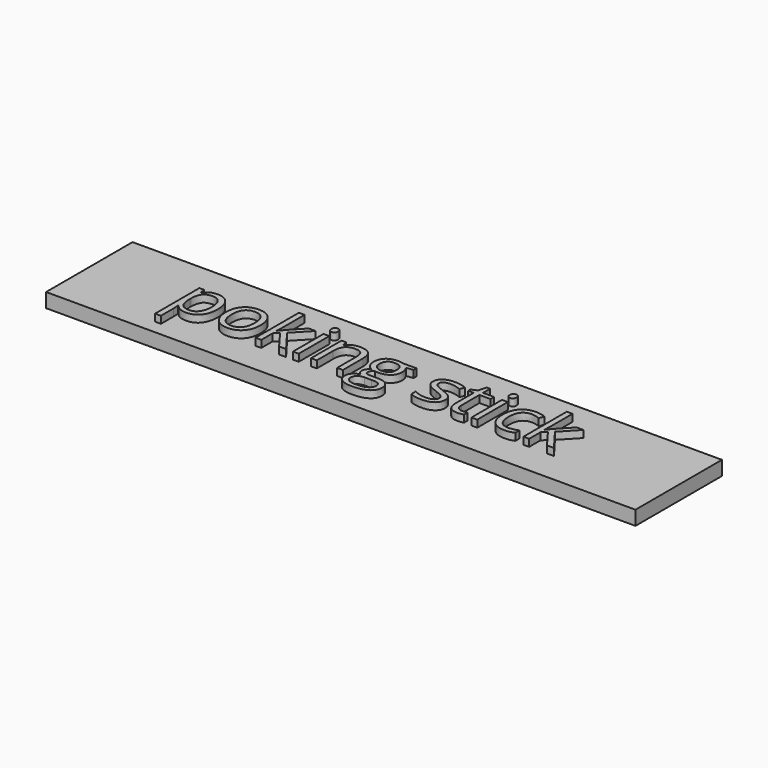
from build123d import *

# Parameters (mm, degrees)
F0_W         = 105.0174571574
F0_H         = 19.2578183487
F0_W_2       = 1.0298908098
F0_H_2       = 6.7964855942
F1_DEPTH     = 2.54
F0_TEXT_SIZE = 12.7000022783
F2_DEPTH     = 3.81


# Not quite as in the source:
# - Text() gives the source's letters only with a copy of the font that has no kerning and outlines rounded to 1/6400 em; it was checked with that copy


with BuildPart() as f1:
    # F0 (on Top) → F1 (new body)
    with BuildSketch(Plane.XY):
        with Locations((9.0054553002, 18.7729089521)):
            Rectangle(F0_W, F0_H)
        with BuildLine():
            add(Edge.make_bspline(
                [(-20.8257423863, 15.4884978257), (-21.5728597078, 14.5608023468), (-22.900406821, 14.5608023468)],
                knots=[0, 0, 0, 1, 1, 1], degree=2))
            add(Edge.make_bspline(
                [(-22.900406821, 14.5608023468), (-23.5651725652, 14.5608023468), (-24.1138523511, 14.8058727032)],
                knots=[0, 0, 0, 1, 1, 1], degree=2))
            add(Edge.make_bspline(
                [(-24.1138523511, 14.8058727032), (-24.6625321371, 15.0509430597), (-25.0336103286, 15.5609275262)],
                knots=[0, 0, 0, 1, 1, 1], degree=2))
            Line((-25.0336103286, 15.5609275262), (-25.1090165922, 15.5609275262))
            add(Edge.make_bspline(
                [(-25.1090165922, 15.5609275262), (-25.0336103286, 14.9656149194), (-25.0336103286, 14.4318179486)],
                knots=[0, 0, 0, 1, 1, 1], degree=2))
            Line((-25.0336103286, 14.4318179486), (-25.0336103286, 11.6338486967))
            Line((-25.0336103286, 11.6338486967), (-26.0635011384, 11.6338486967))
            Line((-26.0635011384, 11.6338486967), (-26.0635011384, 21.4823035884))
            Line((-26.0635011384, 21.4823035884), (-25.2260947382, 21.4823035884))
            Line((-25.2260947382, 21.4823035884), (-25.0832197125, 20.5516315465))
            Line((-25.0832197125, 20.5516315465), (-25.0336103286, 20.5516315465))
            add(Edge.make_bspline(
                [(-25.0336103286, 20.5516315465), (-24.6367352574, 21.1112253969), (-24.1098836004, 21.3592723164)],
                knots=[0, 0, 0, 1, 1, 1], degree=2))
            add(Edge.make_bspline(
                [(-24.1098836004, 21.3592723164), (-23.5830319434, 21.6073192359), (-22.900406821, 21.6073192359)],
                knots=[0, 0, 0, 1, 1, 1], degree=2))
            add(Edge.make_bspline(
                [(-22.900406821, 21.6073192359), (-21.5490472035, 21.6073192359), (-20.8138361341, 20.68260032)],
                knots=[0, 0, 0, 1, 1, 1], degree=2))
            add(Edge.make_bspline(
                [(-20.8138361341, 20.68260032), (-20.0786250647, 19.7578814041), (-20.0786250647, 18.091006105)],
                knots=[0, 0, 0, 1, 1, 1], degree=2))
            add(Edge.make_bspline(
                [(-20.0786250647, 18.091006105), (-20.0786250647, 16.4161933046), (-20.8257423863, 15.4884978257)],
                knots=[0, 0, 0, 1, 1, 1], degree=2))
        make_face(mode=Mode.SUBTRACT)
        with BuildLine():
            add(Edge.make_bspline(
                [(-13.2553504032, 20.657795628), (-12.4149674399, 19.7082720202), (-12.4149674399, 18.091006105)],
                knots=[0, 0, 0, 1, 1, 1], degree=2))
            add(Edge.make_bspline(
                [(-12.4149674399, 18.091006105), (-12.4149674399, 16.4280995567), (-13.2513816525, 15.4944509517)],
                knots=[0, 0, 0, 1, 1, 1], degree=2))
            add(Edge.make_bspline(
                [(-13.2513816525, 15.4944509517), (-14.087795865, 14.5608023468), (-15.5641711299, 14.5608023468)],
                knots=[0, 0, 0, 1, 1, 1], degree=2))
            add(Edge.make_bspline(
                [(-15.5641711299, 14.5608023468), (-16.4769837936, 14.5608023468), (-17.1834214204, 14.9894274236)],
                knots=[0, 0, 0, 1, 1, 1], degree=2))
            add(Edge.make_bspline(
                [(-17.1834214204, 14.9894274236), (-17.8898590471, 15.4180525005), (-18.2748278662, 16.217755769)],
                knots=[0, 0, 0, 1, 1, 1], degree=2))
            add(Edge.make_bspline(
                [(-18.2748278662, 16.217755769), (-18.6597966852, 17.0174590375), (-18.6597966852, 18.091006105)],
                knots=[0, 0, 0, 1, 1, 1], degree=2))
            add(Edge.make_bspline(
                [(-18.6597966852, 18.091006105), (-18.6597966852, 19.751928278), (-17.8283434111, 20.6796237569)],
                knots=[0, 0, 0, 1, 1, 1], degree=2))
            add(Edge.make_bspline(
                [(-17.8283434111, 20.6796237569), (-16.9968901369, 21.6073192359), (-15.520514872, 21.6073192359)],
                knots=[0, 0, 0, 1, 1, 1], degree=2))
            add(Edge.make_bspline(
                [(-15.520514872, 21.6073192359), (-14.0957333665, 21.6073192359), (-13.2553504032, 20.657795628)],
                knots=[0, 0, 0, 1, 1, 1], degree=2))
        make_face(mode=Mode.SUBTRACT)
        with Locations((-3.4287236404, 18.0840607913)):
            Rectangle(F0_W_2, F0_H_2, mode=Mode.SUBTRACT)
        with BuildLine():
            Line((4.9503013003, 14.6858179942), (3.9204104905, 14.6858179942))
            Line((3.9204104905, 14.6858179942), (3.9204104905, 19.083193783))
            add(Edge.make_bspline(
                [(3.9204104905, 19.083193783), (3.9204104905, 19.9126626818), (3.5423869852, 20.3224361929)],
                knots=[0, 0, 0, 1, 1, 1], degree=2))
            add(Edge.make_bspline(
                [(3.5423869852, 20.3224361929), (3.1643634799, 20.7322097039), (2.35672271, 20.7322097039)],
                knots=[0, 0, 0, 1, 1, 1], degree=2))
            add(Edge.make_bspline(
                [(2.35672271, 20.7322097039), (1.2911131439, 20.7322097039), (0.7950193049, 20.155748663)],
                knots=[0, 0, 0, 1, 1, 1], degree=2))
            add(Edge.make_bspline(
                [(0.7950193049, 20.155748663), (0.2989254659, 19.579287622), (0.2989254659, 18.2517405089)],
                knots=[0, 0, 0, 1, 1, 1], degree=2))
            Line((0.2989254659, 18.2517405089), (0.2989254659, 14.6858179942))
            Line((0.2989254659, 14.6858179942), (-0.7309653439, 14.6858179942))
            Line((-0.7309653439, 14.6858179942), (-0.7309653439, 21.4823035884))
            Line((-0.7309653439, 21.4823035884), (0.1064410563, 21.4823035884))
            Line((0.1064410563, 21.4823035884), (0.2731285862, 20.5516315465))
            Line((0.2731285862, 20.5516315465), (0.3227379701, 20.5516315465))
            add(Edge.make_bspline(
                [(0.3227379701, 20.5516315465), (0.6402380271, 21.0536785115), (1.2107459419, 21.3304988737)],
                knots=[0, 0, 0, 1, 1, 1], degree=2))
            add(Edge.make_bspline(
                [(1.2107459419, 21.3304988737), (1.7812538568, 21.6073192359), (2.4817383574, 21.6073192359)],
                knots=[0, 0, 0, 1, 1, 1], degree=2))
            add(Edge.make_bspline(
                [(2.4817383574, 21.6073192359), (3.7100667028, 21.6073192359), (4.3301840015, 21.0149831921)],
                knots=[0, 0, 0, 1, 1, 1], degree=2))
            add(Edge.make_bspline(
                [(4.3301840015, 21.0149831921), (4.9503013003, 20.4226471483), (4.9503013003, 19.1189125394)],
                knots=[0, 0, 0, 1, 1, 1], degree=2))
            Line((4.9503013003, 19.1189125394), (4.9503013003, 14.6858179942))
        make_face(mode=Mode.SUBTRACT)
        with BuildLine():
            Line((10.2763647558, 21.4823035884), (12.6258651772, 21.4823035884))
            Line((12.6258651772, 21.4823035884), (12.6258651772, 20.8314284717))
            Line((12.6258651772, 20.8314284717), (11.3677712015, 20.68260032))
            add(Edge.make_bspline(
                [(11.3677712015, 20.68260032), (11.5404118575, 20.4663034062), (11.6773337571, 20.1150689682)],
                knots=[0, 0, 0, 1, 1, 1], degree=2))
            add(Edge.make_bspline(
                [(11.6773337571, 20.1150689682), (11.8142556566, 19.7638345301), (11.8142556566, 19.3252875765)],
                knots=[0, 0, 0, 1, 1, 1], degree=2))
            add(Edge.make_bspline(
                [(11.8142556566, 19.3252875765), (11.8142556566, 18.3251623971), (11.1316305342, 17.7298497903)],
                knots=[0, 0, 0, 1, 1, 1], degree=2))
            add(Edge.make_bspline(
                [(11.1316305342, 17.7298497903), (10.4490054117, 17.1345371835), (9.2583801981, 17.1345371835)],
                knots=[0, 0, 0, 1, 1, 1], degree=2))
            add(Edge.make_bspline(
                [(9.2583801981, 17.1345371835), (8.9547707687, 17.1345371835), (8.688864471, 17.1841465674)],
                knots=[0, 0, 0, 1, 1, 1], degree=2))
            add(Edge.make_bspline(
                [(8.688864471, 17.1841465674), (8.0320362281, 16.8368808801), (8.0320362281, 16.3110214107)],
                knots=[0, 0, 0, 1, 1, 1], degree=2))
            add(Edge.make_bspline(
                [(8.0320362281, 16.3110214107), (8.0320362281, 16.0312244855), (8.2612315818, 15.8982713367)],
                knots=[0, 0, 0, 1, 1, 1], degree=2))
            add(Edge.make_bspline(
                [(8.2612315818, 15.8982713367), (8.4904269354, 15.7653181878), (9.0480364104, 15.7653181878)],
                knots=[0, 0, 0, 1, 1, 1], degree=2))
            Line((9.0480364104, 15.7653181878), (10.2505678761, 15.7653181878))
            add(Edge.make_bspline(
                [(10.2505678761, 15.7653181878), (11.3558649494, 15.7653181878), (11.9472088055, 15.2999821669)],
                knots=[0, 0, 0, 1, 1, 1], degree=2))
            add(Edge.make_bspline(
                [(11.9472088055, 15.2999821669), (12.5385526616, 14.8346461459), (12.5385526616, 13.9476303618)],
                knots=[0, 0, 0, 1, 1, 1], degree=2))
            add(Edge.make_bspline(
                [(12.5385526616, 13.9476303618), (12.5385526616, 12.8185207842), (11.6336774993, 12.2261847404)],
                knots=[0, 0, 0, 1, 1, 1], degree=2))
            add(Edge.make_bspline(
                [(11.6336774993, 12.2261847404), (10.7288023369, 11.6338486967), (8.9924739004, 11.6338486967)],
                knots=[0, 0, 0, 1, 1, 1], degree=2))
            add(Edge.make_bspline(
                [(8.9924739004, 11.6338486967), (7.6589736612, 11.6338486967), (6.9366610316, 12.1299425357)],
                knots=[0, 0, 0, 1, 1, 1], degree=2))
            add(Edge.make_bspline(
                [(6.9366610316, 12.1299425357), (6.2143484021, 12.6260363747), (6.2143484021, 13.5328959123)],
                knots=[0, 0, 0, 1, 1, 1], degree=2))
            add(Edge.make_bspline(
                [(6.2143484021, 13.5328959123), (6.2143484021, 14.1520210234), (6.6112234733, 14.6054507923)],
                knots=[0, 0, 0, 1, 1, 1], degree=2))
            add(Edge.make_bspline(
                [(6.6112234733, 14.6054507923), (7.0080985444, 15.0588805611), (7.7264424233, 15.2196149649)],
                knots=[0, 0, 0, 1, 1, 1], degree=2))
            add(Edge.make_bspline(
                [(7.7264424233, 15.2196149649), (7.4664892517, 15.3366931109), (7.289879845, 15.5847400304)],
                knots=[0, 0, 0, 1, 1, 1], degree=2))
            add(Edge.make_bspline(
                [(7.289879845, 15.5847400304), (7.1132704383, 15.8327869499), (7.1132704383, 16.162193259)],
                knots=[0, 0, 0, 1, 1, 1], degree=2))
            add(Edge.make_bspline(
                [(7.1132704383, 16.162193259), (7.1132704383, 16.5332714506), (7.3117079739, 16.8130683758)],
                knots=[0, 0, 0, 1, 1, 1], degree=2))
            add(Edge.make_bspline(
                [(7.3117079739, 16.8130683758), (7.5101455095, 17.092865301), (7.9387705864, 17.3528184726)],
                knots=[0, 0, 0, 1, 1, 1], degree=2))
            add(Edge.make_bspline(
                [(7.9387705864, 17.3528184726), (7.4109267417, 17.5691153864), (7.0795360573, 18.0900139174)],
                knots=[0, 0, 0, 1, 1, 1], degree=2))
            add(Edge.make_bspline(
                [(7.0795360573, 18.0900139174), (6.7481453728, 18.6109124483), (6.7481453728, 19.2816313186)],
                knots=[0, 0, 0, 1, 1, 1], degree=2))
            add(Edge.make_bspline(
                [(6.7481453728, 19.2816313186), (6.7481453728, 20.3968502687), (7.4178720555, 21.0020847523)],
                knots=[0, 0, 0, 1, 1, 1], degree=2))
            add(Edge.make_bspline(
                [(7.4178720555, 21.0020847523), (8.0875987381, 21.6073192359), (9.3139427081, 21.6073192359)],
                knots=[0, 0, 0, 1, 1, 1], degree=2))
            add(Edge.make_bspline(
                [(9.3139427081, 21.6073192359), (9.8477396789, 21.6073192359), (10.2763647558, 21.4823035884)],
                knots=[0, 0, 0, 1, 1, 1], degree=2))
        make_face(mode=Mode.SUBTRACT)
        with BuildLine():
            add(Edge.make_bspline(
                [(21.2797261047, 17.6623810282), (21.7043824309, 17.2158965731), (21.7043824309, 16.5392245767)],
                knots=[0, 0, 0, 1, 1, 1], degree=2))
            add(Edge.make_bspline(
                [(21.7043824309, 16.5392245767), (21.7043824309, 15.5906931565), (20.9979448041, 15.0757477516)],
                knots=[0, 0, 0, 1, 1, 1], degree=2))
            add(Edge.make_bspline(
                [(20.9979448041, 15.0757477516), (20.2915071774, 14.5608023468), (19.0135694482, 14.5608023468)],
                knots=[0, 0, 0, 1, 1, 1], degree=2))
            add(Edge.make_bspline(
                [(19.0135694482, 14.5608023468), (17.6622098307, 14.5608023468), (16.9061628201, 14.9894274236)],
                knots=[0, 0, 0, 1, 1, 1], degree=2))
            Line((16.9061628201, 14.9894274236), (16.9061628201, 15.9439119699))
            add(Edge.make_bspline(
                [(16.9061628201, 15.9439119699), (17.396303533, 15.6958650504), (17.9568895711, 15.5539822124)],
                knots=[0, 0, 0, 1, 1, 1], degree=2))
            add(Edge.make_bspline(
                [(17.9568895711, 15.5539822124), (18.5174756092, 15.4120993745), (19.0393663278, 15.4120993745)],
                knots=[0, 0, 0, 1, 1, 1], degree=2))
            add(Edge.make_bspline(
                [(19.0393663278, 15.4120993745), (19.8450227223, 15.4120993745), (20.2786087376, 15.6690759831)],
                knots=[0, 0, 0, 1, 1, 1], degree=2))
            add(Edge.make_bspline(
                [(20.2786087376, 15.6690759831), (20.7121947529, 15.9260525917), (20.7121947529, 16.4538964364)],
                knots=[0, 0, 0, 1, 1, 1], degree=2))
            add(Edge.make_bspline(
                [(20.7121947529, 16.4538964364), (20.7121947529, 16.8507715076), (20.3688978163, 17.1325528081)],
                knots=[0, 0, 0, 1, 1, 1], degree=2))
            add(Edge.make_bspline(
                [(20.3688978163, 17.1325528081), (20.0256008797, 17.4143341087), (19.0254757003, 17.7993029277)],
                knots=[0, 0, 0, 1, 1, 1], degree=2))
            add(Edge.make_bspline(
                [(19.0254757003, 17.7993029277), (18.0769442801, 18.1525217411), (17.6770926459, 18.4164436634)],
                knots=[0, 0, 0, 1, 1, 1], degree=2))
            add(Edge.make_bspline(
                [(17.6770926459, 18.4164436634), (17.2772410117, 18.6803655858), (17.0817800391, 19.0147328333)],
                knots=[0, 0, 0, 1, 1, 1], degree=2))
            add(Edge.make_bspline(
                [(17.0817800391, 19.0147328333), (16.8863190665, 19.3491000807), (16.8863190665, 19.813443914)],
                knots=[0, 0, 0, 1, 1, 1], degree=2))
            add(Edge.make_bspline(
                [(16.8863190665, 19.813443914), (16.8863190665, 20.6448971882), (17.5629910629, 21.126108212)],
                knots=[0, 0, 0, 1, 1, 1], degree=2))
            add(Edge.make_bspline(
                [(17.5629910629, 21.126108212), (18.2396630593, 21.6073192359), (19.4163976454, 21.6073192359)],
                knots=[0, 0, 0, 1, 1, 1], degree=2))
            add(Edge.make_bspline(
                [(19.4163976454, 21.6073192359), (20.5137572173, 21.6073192359), (21.5634917806, 21.1608347808)],
                knots=[0, 0, 0, 1, 1, 1], degree=2))
            Line((21.5634917806, 21.1608347808), (21.1963823397, 20.3234283805))
            add(Edge.make_bspline(
                [(21.1963823397, 20.3234283805), (20.1744290314, 20.744115956), (19.3429757573, 20.744115956)],
                knots=[0, 0, 0, 1, 1, 1], degree=2))
            add(Edge.make_bspline(
                [(19.3429757573, 20.744115956), (18.6107412509, 20.744115956), (18.2386708716, 20.5149206024)],
                knots=[0, 0, 0, 1, 1, 1], degree=2))
            add(Edge.make_bspline(
                [(18.2386708716, 20.5149206024), (17.8666004924, 20.2857252488), (17.8666004924, 19.8828970515)],
                knots=[0, 0, 0, 1, 1, 1], degree=2))
            add(Edge.make_bspline(
                [(17.8666004924, 19.8828970515), (17.8666004924, 19.6090532524), (18.006498955, 19.4175610305)],
                knots=[0, 0, 0, 1, 1, 1], degree=2))
            add(Edge.make_bspline(
                [(18.006498955, 19.4175610305), (18.1463974176, 19.2260688087), (18.4559599731, 19.052435965)],
                knots=[0, 0, 0, 1, 1, 1], degree=2))
            add(Edge.make_bspline(
                [(18.4559599731, 19.052435965), (18.7655225287, 18.8788031214), (19.6465851867, 18.5493968123)],
                knots=[0, 0, 0, 1, 1, 1], degree=2))
            add(Edge.make_bspline(
                [(19.6465851867, 18.5493968123), (20.8550697785, 18.1088654833), (21.2797261047, 17.6623810282)],
                knots=[0, 0, 0, 1, 1, 1], degree=2))
        make_face(mode=Mode.SUBTRACT)
        with Locations((28.3768445654, 18.0840607913)):
            Rectangle(F0_W_2, F0_H_2, mode=Mode.SUBTRACT)
        with BuildLine():
            add(Edge.make_bspline(
                [(35.5076974071, 14.9160055355), (34.82705666, 14.5608023468), (33.7912127242, 14.5608023468)],
                knots=[0, 0, 0, 1, 1, 1], degree=2))
            add(Edge.make_bspline(
                [(33.7912127242, 14.5608023468), (32.3148374593, 14.5608023468), (31.5052123141, 15.4696462598)],
                knots=[0, 0, 0, 1, 1, 1], degree=2))
            add(Edge.make_bspline(
                [(31.5052123141, 15.4696462598), (30.6955871688, 16.3784901728), (30.6955871688, 18.0413967211)],
                knots=[0, 0, 0, 1, 1, 1], degree=2))
            add(Edge.make_bspline(
                [(30.6955871688, 18.0413967211), (30.6955871688, 19.7459751519), (31.5181107539, 20.6766471939)],
                knots=[0, 0, 0, 1, 1, 1], degree=2))
            add(Edge.make_bspline(
                [(31.5181107539, 20.6766471939), (32.340634339, 21.6073192359), (33.8586814863, 21.6073192359)],
                knots=[0, 0, 0, 1, 1, 1], degree=2))
            add(Edge.make_bspline(
                [(33.8586814863, 21.6073192359), (34.3488221992, 21.6073192359), (34.8389629121, 21.5011551543)],
                knots=[0, 0, 0, 1, 1, 1], degree=2))
            add(Edge.make_bspline(
                [(34.8389629121, 21.5011551543), (35.3291036251, 21.3949910728), (35.6069161749, 21.2521160471)],
                knots=[0, 0, 0, 1, 1, 1], degree=2))
            Line((35.6069161749, 21.2521160471), (35.2914004933, 20.3789908905))
            add(Edge.make_bspline(
                [(35.2914004933, 20.3789908905), (34.9500879321, 20.5159127901), (34.5472597348, 20.6052096811)],
                knots=[0, 0, 0, 1, 1, 1], degree=2))
            add(Edge.make_bspline(
                [(34.5472597348, 20.6052096811), (34.1444315375, 20.6945065721), (33.834868982, 20.6945065721)],
                knots=[0, 0, 0, 1, 1, 1], degree=2))
            add(Edge.make_bspline(
                [(33.834868982, 20.6945065721), (31.7631811104, 20.6945065721), (31.7631811104, 18.0533029733)],
                knots=[0, 0, 0, 1, 1, 1], degree=2))
            add(Edge.make_bspline(
                [(31.7631811104, 18.0533029733), (31.7631811104, 16.8011621237), (32.2682046385, 16.131435441)],
                knots=[0, 0, 0, 1, 1, 1], degree=2))
            add(Edge.make_bspline(
                [(32.2682046385, 16.131435441), (32.7732281666, 15.4617087584), (33.7654158446, 15.4617087584)],
                knots=[0, 0, 0, 1, 1, 1], degree=2))
            add(Edge.make_bspline(
                [(33.7654158446, 15.4617087584), (34.6147284969, 15.4617087584), (35.5076974071, 15.8268338239)],
                knots=[0, 0, 0, 1, 1, 1], degree=2))
            Line((35.5076974071, 15.8268338239), (35.5076974071, 14.9160055355))
        make_face(mode=Mode.SUBTRACT)
        with BuildLine():
            Line((-9.6408106923, 18.1644279932), (-9.5912013084, 18.1644279932))
            add(Edge.make_bspline(
                [(-9.5912013084, 18.1644279932), (-9.3252950107, 18.5434436862), (-8.7795917878, 19.1566156712)],
                knots=[0, 0, 0, 1, 1, 1], degree=2))
            Line((-8.7795917878, 19.1566156712), (-6.584872644, 21.4823035884))
            Line((-6.584872644, 21.4823035884), (-5.3624974248, 21.4823035884))
            Line((-5.3624974248, 21.4823035884), (-8.1168104189, 18.587099944))
            Line((-8.1168104189, 18.587099944), (-5.1700130152, 14.6858179942))
            Line((-5.1700130152, 14.6858179942), (-6.4162007388, 14.6858179942))
            Line((-6.4162007388, 14.6858179942), (-8.8172949195, 17.8985216955))
            Line((-8.8172949195, 17.8985216955), (-9.5912013084, 17.2278028252))
            Line((-9.5912013084, 17.2278028252), (-9.5912013084, 14.6858179942))
            Line((-9.5912013084, 14.6858179942), (-10.609185866, 14.6858179942))
            Line((-10.609185866, 14.6858179942), (-10.609185866, 24.3358353503))
            Line((-10.609185866, 24.3358353503), (-9.5912013084, 24.3358353503))
            Line((-9.5912013084, 24.3358353503), (-9.5912013084, 19.2181313072))
            add(Edge.make_bspline(
                [(-9.5912013084, 19.2181313072), (-9.5912013084, 18.8788031214), (-9.6408106923, 18.1644279932)],
                knots=[0, 0, 0, 1, 1, 1], degree=2))
        make_face(mode=Mode.SUBTRACT)
        with BuildLine():
            add(Edge.make_bspline(
                [(-3.8573487172, 22.8058819509), (-4.0309815609, 22.9765382315), (-4.0309815609, 23.3238039188)],
                knots=[0, 0, 0, 1, 1, 1], degree=2))
            add(Edge.make_bspline(
                [(-4.0309815609, 23.3238039188), (-4.0309815609, 23.6770227321), (-3.8573487172, 23.8417258867)],
                knots=[0, 0, 0, 1, 1, 1], degree=2))
            add(Edge.make_bspline(
                [(-3.8573487172, 23.8417258867), (-3.6837158736, 24.0064290412), (-3.4217783266, 24.0064290412)],
                knots=[0, 0, 0, 1, 1, 1], degree=2))
            add(Edge.make_bspline(
                [(-3.4217783266, 24.0064290412), (-3.1737314071, 24.0064290412), (-2.9941454374, 23.8387493237)],
                knots=[0, 0, 0, 1, 1, 1], degree=2))
            add(Edge.make_bspline(
                [(-2.9941454374, 23.8387493237), (-2.8145594677, 23.6710696061), (-2.8145594677, 23.3238039188)],
                knots=[0, 0, 0, 1, 1, 1], degree=2))
            add(Edge.make_bspline(
                [(-2.8145594677, 23.3238039188), (-2.8145594677, 22.9765382315), (-2.9941454374, 22.8058819509)],
                knots=[0, 0, 0, 1, 1, 1], degree=2))
            add(Edge.make_bspline(
                [(-2.9941454374, 22.8058819509), (-3.1737314071, 22.6352256703), (-3.4217783266, 22.6352256703)],
                knots=[0, 0, 0, 1, 1, 1], degree=2))
            add(Edge.make_bspline(
                [(-3.4217783266, 22.6352256703), (-3.6837158736, 22.6352256703), (-3.8573487172, 22.8058819509)],
                knots=[0, 0, 0, 1, 1, 1], degree=2))
        make_face(mode=Mode.SUBTRACT)
        with BuildLine():
            add(Edge.make_bspline(
                [(24.7742111066, 15.7405134959), (25.0659142839, 15.4120993745), (25.573914375, 15.4120993745)],
                knots=[0, 0, 0, 1, 1, 1], degree=2))
            add(Edge.make_bspline(
                [(25.573914375, 15.4120993745), (25.8477581742, 15.4120993745), (26.1017582197, 15.4517868816)],
                knots=[0, 0, 0, 1, 1, 1], degree=2))
            add(Edge.make_bspline(
                [(26.1017582197, 15.4517868816), (26.3557582653, 15.4914743887), (26.504586417, 15.5351306465)],
                knots=[0, 0, 0, 1, 1, 1], degree=2))
            Line((26.504586417, 15.5351306465), (26.504586417, 14.7473336302))
            add(Edge.make_bspline(
                [(26.504586417, 14.7473336302), (26.3378988871, 14.667958616), (26.0124613287, 14.6143804814)],
                knots=[0, 0, 0, 1, 1, 1], degree=2))
            add(Edge.make_bspline(
                [(26.0124613287, 14.6143804814), (25.6870237703, 14.5608023468), (25.4250862233, 14.5608023468)],
                knots=[0, 0, 0, 1, 1, 1], degree=2))
            add(Edge.make_bspline(
                [(25.4250862233, 14.5608023468), (23.4546014949, 14.5608023468), (23.4546014949, 16.6384433445)],
                knots=[0, 0, 0, 1, 1, 1], degree=2))
            Line((23.4546014949, 16.6384433445), (23.4546014949, 20.68260032))
            Line((23.4546014949, 20.68260032), (22.4802731951, 20.68260032))
            Line((22.4802731951, 20.68260032), (22.4802731951, 21.178694159))
            Line((22.4802731951, 21.178694159), (23.4546014949, 21.6073192359))
            Line((23.4546014949, 21.6073192359), (23.8871953225, 23.0578976211))
            Line((23.8871953225, 23.0578976211), (24.4825079293, 23.0578976211))
            Line((24.4825079293, 23.0578976211), (24.4825079293, 21.4823035884))
            Line((24.4825079293, 21.4823035884), (26.4549770331, 21.4823035884))
            Line((26.4549770331, 21.4823035884), (26.4549770331, 20.68260032))
            Line((26.4549770331, 20.68260032), (24.4825079293, 20.68260032))
            Line((24.4825079293, 20.68260032), (24.4825079293, 16.6820996023))
            add(Edge.make_bspline(
                [(24.4825079293, 16.6820996023), (24.4825079293, 16.0689276173), (24.7742111066, 15.7405134959)],
                knots=[0, 0, 0, 1, 1, 1], degree=2))
        make_face(mode=Mode.SUBTRACT)
        with BuildLine():
            add(Edge.make_bspline(
                [(27.9482194885, 22.8058819509), (27.7745866448, 22.9765382315), (27.7745866448, 23.3238039188)],
                knots=[0, 0, 0, 1, 1, 1], degree=2))
            add(Edge.make_bspline(
                [(27.7745866448, 23.3238039188), (27.7745866448, 23.6770227321), (27.9482194885, 23.8417258867)],
                knots=[0, 0, 0, 1, 1, 1], degree=2))
            add(Edge.make_bspline(
                [(27.9482194885, 23.8417258867), (28.1218523321, 24.0064290412), (28.3837898791, 24.0064290412)],
                knots=[0, 0, 0, 1, 1, 1], degree=2))
            add(Edge.make_bspline(
                [(28.3837898791, 24.0064290412), (28.6318367986, 24.0064290412), (28.8114227683, 23.8387493237)],
                knots=[0, 0, 0, 1, 1, 1], degree=2))
            add(Edge.make_bspline(
                [(28.8114227683, 23.8387493237), (28.9910087381, 23.6710696061), (28.9910087381, 23.3238039188)],
                knots=[0, 0, 0, 1, 1, 1], degree=2))
            add(Edge.make_bspline(
                [(28.9910087381, 23.3238039188), (28.9910087381, 22.9765382315), (28.8114227683, 22.8058819509)],
                knots=[0, 0, 0, 1, 1, 1], degree=2))
            add(Edge.make_bspline(
                [(28.8114227683, 22.8058819509), (28.6318367986, 22.6352256703), (28.3837898791, 22.6352256703)],
                knots=[0, 0, 0, 1, 1, 1], degree=2))
            add(Edge.make_bspline(
                [(28.3837898791, 22.6352256703), (28.1218523321, 22.6352256703), (27.9482194885, 22.8058819509)],
                knots=[0, 0, 0, 1, 1, 1], degree=2))
        make_face(mode=Mode.SUBTRACT)
        with BuildLine():
            Line((38.0893697452, 18.1644279932), (38.1389791291, 18.1644279932))
            add(Edge.make_bspline(
                [(38.1389791291, 18.1644279932), (38.4048854268, 18.5434436862), (38.9505886497, 19.1566156712)],
                knots=[0, 0, 0, 1, 1, 1], degree=2))
            Line((38.9505886497, 19.1566156712), (41.1453077935, 21.4823035884))
            Line((41.1453077935, 21.4823035884), (42.3676830127, 21.4823035884))
            Line((42.3676830127, 21.4823035884), (39.6133700186, 18.587099944))
            Line((39.6133700186, 18.587099944), (42.5601674223, 14.6858179942))
            Line((42.5601674223, 14.6858179942), (41.3139796987, 14.6858179942))
            Line((41.3139796987, 14.6858179942), (38.912885518, 17.8985216955))
            Line((38.912885518, 17.8985216955), (38.1389791291, 17.2278028252))
            Line((38.1389791291, 17.2278028252), (38.1389791291, 14.6858179942))
            Line((38.1389791291, 14.6858179942), (37.1209945715, 14.6858179942))
            Line((37.1209945715, 14.6858179942), (37.1209945715, 24.3358353503))
            Line((37.1209945715, 24.3358353503), (38.1389791291, 24.3358353503))
            Line((38.1389791291, 24.3358353503), (38.1389791291, 19.2181313072))
            add(Edge.make_bspline(
                [(38.1389791291, 19.2181313072), (38.1389791291, 18.8788031214), (38.0893697452, 18.1644279932)],
                knots=[0, 0, 0, 1, 1, 1], degree=2))
        make_face(mode=Mode.SUBTRACT)
    extrude(amount=F1_DEPTH)

    # F0 (on Top) → F2 (join)
    with BuildSketch(Plane.XY):
        with Locations((-27.1549075842, 14.6858179942)):
            Text('poking stick', F0_TEXT_SIZE, font='Open Sans', text_align=(TextAlign.LEFT, TextAlign.BOTTOM))
    extrude(amount=F2_DEPTH)


with BuildPart() as f1b:
    # F0 (on Top) → F1, piece 2 (new body)
    with BuildSketch(Plane.XY):
        with BuildLine():
            add(Edge.make_bspline(
                [(-21.6452894083, 20.0535533321), (-22.1443598103, 20.7322097039), (-23.0492349727, 20.7322097039)],
                knots=[0, 0, 0, 1, 1, 1], degree=2))
            add(Edge.make_bspline(
                [(-23.0492349727, 20.7322097039), (-24.0910320345, 20.7322097039), (-24.5563680555, 20.155748663)],
                knots=[0, 0, 0, 1, 1, 1], degree=2))
            add(Edge.make_bspline(
                [(-24.5563680555, 20.155748663), (-25.0217040765, 19.579287622), (-25.0336103286, 18.319209271)],
                knots=[0, 0, 0, 1, 1, 1], degree=2))
            Line((-25.0336103286, 18.319209271), (-25.0336103286, 18.091006105))
            add(Edge.make_bspline(
                [(-25.0336103286, 18.091006105), (-25.0336103286, 16.658287098), (-24.5563680555, 16.0411463623)],
                knots=[0, 0, 0, 1, 1, 1], degree=2))
            add(Edge.make_bspline(
                [(-24.5563680555, 16.0411463623), (-24.0791257824, 15.4240056266), (-23.0254224684, 15.4240056266)],
                knots=[0, 0, 0, 1, 1, 1], degree=2))
            add(Edge.make_bspline(
                [(-23.0254224684, 15.4240056266), (-22.1443598103, 15.4240056266), (-21.6452894083, 16.1373885671)],
                knots=[0, 0, 0, 1, 1, 1], degree=2))
            add(Edge.make_bspline(
                [(-21.6452894083, 16.1373885671), (-21.1462190063, 16.8507715076), (-21.1462190063, 18.1029123572)],
                knots=[0, 0, 0, 1, 1, 1], degree=2))
            add(Edge.make_bspline(
                [(-21.1462190063, 18.1029123572), (-21.1462190063, 19.3748969604), (-21.6452894083, 20.0535533321)],
                knots=[0, 0, 0, 1, 1, 1], degree=2))
        make_face()
    extrude(amount=F1_DEPTH)


with BuildPart() as f1c:
    # F0 (on Top) → F1, piece 3 (new body)
    with BuildSketch(Plane.XY):
        with BuildLine():
            add(Edge.make_bspline(
                [(-17.0772573388, 20.0684361473), (-17.5922027437, 19.4046625907), (-17.5922027437, 18.091006105)],
                knots=[0, 0, 0, 1, 1, 1], degree=2))
            add(Edge.make_bspline(
                [(-17.5922027437, 18.091006105), (-17.5922027437, 16.7872714962), (-17.0713042128, 16.1056385614)],
                knots=[0, 0, 0, 1, 1, 1], degree=2))
            add(Edge.make_bspline(
                [(-17.0713042128, 16.1056385614), (-16.5504056818, 15.4240056266), (-15.5403586256, 15.4240056266)],
                knots=[0, 0, 0, 1, 1, 1], degree=2))
            add(Edge.make_bspline(
                [(-15.5403586256, 15.4240056266), (-14.5283271941, 15.4240056266), (-14.0044521001, 16.1026619984)],
                knots=[0, 0, 0, 1, 1, 1], degree=2))
            add(Edge.make_bspline(
                [(-14.0044521001, 16.1026619984), (-13.4805770061, 16.7813183701), (-13.4805770061, 18.091006105)],
                knots=[0, 0, 0, 1, 1, 1], degree=2))
            add(Edge.make_bspline(
                [(-13.4805770061, 18.091006105), (-13.4805770061, 19.3868032125), (-14.0044521001, 20.0595064582)],
                knots=[0, 0, 0, 1, 1, 1], degree=2))
            add(Edge.make_bspline(
                [(-14.0044521001, 20.0595064582), (-14.5283271941, 20.7322097039), (-15.5522648777, 20.7322097039)],
                knots=[0, 0, 0, 1, 1, 1], degree=2))
            add(Edge.make_bspline(
                [(-15.5522648777, 20.7322097039), (-16.5623119339, 20.7322097039), (-17.0772573388, 20.0684361473)],
                knots=[0, 0, 0, 1, 1, 1], degree=2))
        make_face()
    extrude(amount=F1_DEPTH)


with BuildPart() as f1d:
    # F0 (on Top) → F1, piece 4 (new body)
    with BuildSketch(Plane.XY):
        with BuildLine():
            add(Edge.make_bspline(
                [(8.1550675002, 20.4653112185), (7.7641455551, 20.075381461), (7.7641455551, 19.3054438229)],
                knots=[0, 0, 0, 1, 1, 1], degree=2))
            add(Edge.make_bspline(
                [(7.7641455551, 19.3054438229), (7.7641455551, 18.5930530701), (8.1669737523, 18.2269358169)],
                knots=[0, 0, 0, 1, 1, 1], degree=2))
            add(Edge.make_bspline(
                [(8.1669737523, 18.2269358169), (8.5698019496, 17.8608185638), (9.2901302038, 17.8608185638)],
                knots=[0, 0, 0, 1, 1, 1], degree=2))
            add(Edge.make_bspline(
                [(9.2901302038, 17.8608185638), (10.796271099, 17.8608185638), (10.796271099, 19.3252875765)],
                knots=[0, 0, 0, 1, 1, 1], degree=2))
            add(Edge.make_bspline(
                [(10.796271099, 19.3252875765), (10.796271099, 20.8552409759), (9.2722708256, 20.8552409759)],
                knots=[0, 0, 0, 1, 1, 1], degree=2))
            add(Edge.make_bspline(
                [(9.2722708256, 20.8552409759), (8.5459894453, 20.8552409759), (8.1550675002, 20.4653112185)],
                knots=[0, 0, 0, 1, 1, 1], degree=2))
        make_face()
    extrude(amount=F1_DEPTH)


with BuildPart() as f1e:
    # F0 (on Top) → F1, piece 5 (new body)
    with BuildSketch(Plane.XY):
        with BuildLine():
            add(Edge.make_bspline(
                [(7.5974580252, 14.5062320245), (7.20653608, 14.171864777), (7.20653608, 13.5448021645)],
                knots=[0, 0, 0, 1, 1, 1], degree=2))
            add(Edge.make_bspline(
                [(7.20653608, 13.5448021645), (7.20653608, 12.9931458155), (7.671872101, 12.7073957643)],
                knots=[0, 0, 0, 1, 1, 1], degree=2))
            add(Edge.make_bspline(
                [(7.671872101, 12.7073957643), (8.137208122, 12.421645713), (9.0043801526, 12.421645713)],
                knots=[0, 0, 0, 1, 1, 1], degree=2))
            add(Edge.make_bspline(
                [(9.0043801526, 12.421645713), (10.30017726, 12.421645713), (10.9232711218, 12.8095910951)],
                knots=[0, 0, 0, 1, 1, 1], degree=2))
            add(Edge.make_bspline(
                [(10.9232711218, 12.8095910951), (11.5463649836, 13.1975364772), (11.5463649836, 13.8603178461)],
                knots=[0, 0, 0, 1, 1, 1], degree=2))
            add(Edge.make_bspline(
                [(11.5463649836, 13.8603178461), (11.5463649836, 14.4119741951), (11.20604461, 14.6262867335)],
                knots=[0, 0, 0, 1, 1, 1], degree=2))
            add(Edge.make_bspline(
                [(11.20604461, 14.6262867335), (10.8657242365, 14.8405992719), (9.9231459424, 14.8405992719)],
                knots=[0, 0, 0, 1, 1, 1], degree=2))
            Line((9.9231459424, 14.8405992719), (8.688864471, 14.8405992719))
            add(Edge.make_bspline(
                [(8.688864471, 14.8405992719), (7.9883799703, 14.8405992719), (7.5974580252, 14.5062320245)],
                knots=[0, 0, 0, 1, 1, 1], degree=2))
        make_face()
    extrude(amount=F1_DEPTH)


solid = Compound([f1.part, f1b.part, f1c.part, f1d.part, f1e.part])
